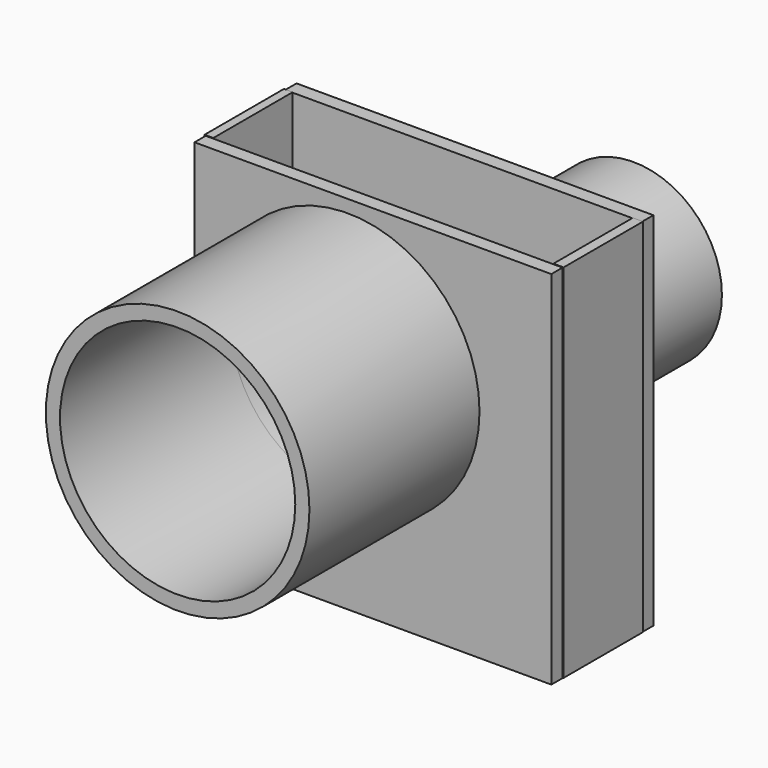
from build123d import *

# Parameters (mm, degrees)
F0_W          = 101.342654407
F0_H          = 102
F0_W_2        = 93.342654407
F0_H_2        = 94
F1_DEPTH      = 28
F2_W          = 3.946882084
F2_H          = 101.9999885866
F3_DEPTH      = 50.4
F3_DEPTH_BACK = 50.3
F2_W_2        = 4
F4_W          = 96
F4_H          = 28
F5_DEPTH      = 96
F7_DEPTH      = 5
F8_R          = 37.2
F8_R_2        = 33.2
F9_DEPTH      = 60
F10_R         = 24.95
F10_R_2       = 20.95
F11_DEPTH     = 60
F12_DEPTH     = 55.8


with BuildPart() as f1:
    # F0 (on Front) → F1 (new body)
    with BuildSketch(Plane.XZ):
        Rectangle(F0_W, F0_H)
        Rectangle(F0_W_2, F0_H_2, mode=Mode.SUBTRACT)
    extrude(amount=F1_DEPTH)

    # F4 (on face) → F5 (cut)
    with BuildSketch(Plane.XY.offset(51)):
        with Locations((-0.1949560344, -14)):
            Rectangle(F4_W, F4_H)
    extrude(amount=-F5_DEPTH, mode=Mode.SUBTRACT)


with BuildPart() as f3:
    # F2 (on Right) → F3 (new body, two sides)
    with BuildSketch(Plane.YZ) as f3_sk:
        with Locations((-30.026558958, -0.1257993281)):
            Rectangle(F2_W, F2_H)
    extrude(amount=F3_DEPTH)
    extrude(f3_sk.sketch, amount=-F3_DEPTH_BACK)

    # F6 (on face) → F7 (cut)
    with BuildSketch(Plane.XZ.offset(32)):
        with BuildLine():
            Line((-7.06, 10.1242063786), (-7.06, 43.3242063786))
            ThreePointArc((-7.06, 43.3242063786), (-30.5359451354, 33.600151514), (-40.26, 10.1242063786))
            Line((-40.26, 10.1242063786), (-7.06, 10.1242063786))
        make_face()
        with BuildLine():
            ThreePointArc((26.14, 10.1242063786), (16.4159451354, 33.600151514), (-7.06, 43.3242063786))
            Line((-7.06, 43.3242063786), (-7.06, 10.1242063786))
            Line((-7.06, 10.1242063786), (26.14, 10.1242063786))
        make_face()
        with BuildLine():
            Line((26.14, 10.1242063786), (-7.06, 10.1242063786))
            Line((-7.06, 10.1242063786), (-7.06, -23.0757936214))
            ThreePointArc((-7.06, -23.0757936214), (16.4159451354, -13.3517387568), (26.14, 10.1242063786))
        make_face()
        with BuildLine():
            Line((-7.06, -23.0757936214), (-7.06, 10.1242063786))
            Line((-7.06, 10.1242063786), (-40.26, 10.1242063786))
            ThreePointArc((-40.26, 10.1242063786), (-30.5359451354, -13.3517387568), (-7.06, -23.0757936214))
        make_face()
    extrude(amount=-F7_DEPTH, mode=Mode.SUBTRACT)

    # F8 (on face) → F9 (join)
    with BuildSketch(Plane.XZ.offset(32)):
        with Locations((-7.06, 10.1242063786)):
            Circle(F8_R)
        with Locations((-7.06, 10.1242063786)):
            Circle(F8_R_2, mode=Mode.SUBTRACT)
    extrude(amount=F9_DEPTH)


with BuildPart() as f3b:
    # F2 (on Right) → F3, piece 2 (new body, two sides)
    with BuildSketch(Plane.YZ) as f3_2_sk:
        with Locations((2, -0.1257993281)):
            Rectangle(F2_W_2, F2_H)
    extrude(amount=F3_DEPTH)
    extrude(f3_2_sk.sketch, amount=-F3_DEPTH_BACK)

    # F10 (on Front) → F11 (join)
    with BuildSketch(Plane.XZ):
        Circle(F10_R)
        Circle(F10_R_2, mode=Mode.SUBTRACT)
    extrude(amount=-F11_DEPTH)

    # F12 (cut): faces of the model
    f12_faces = [f3b.faces().sort_by_distance(p)[0] for p in [
        (0, 4, 0),
        (0, 4, 0),
    ]]
    extrude(f12_faces, amount=-F12_DEPTH, mode=Mode.SUBTRACT)


solid = Compound([f1.part, f3.part, f3b.part])
